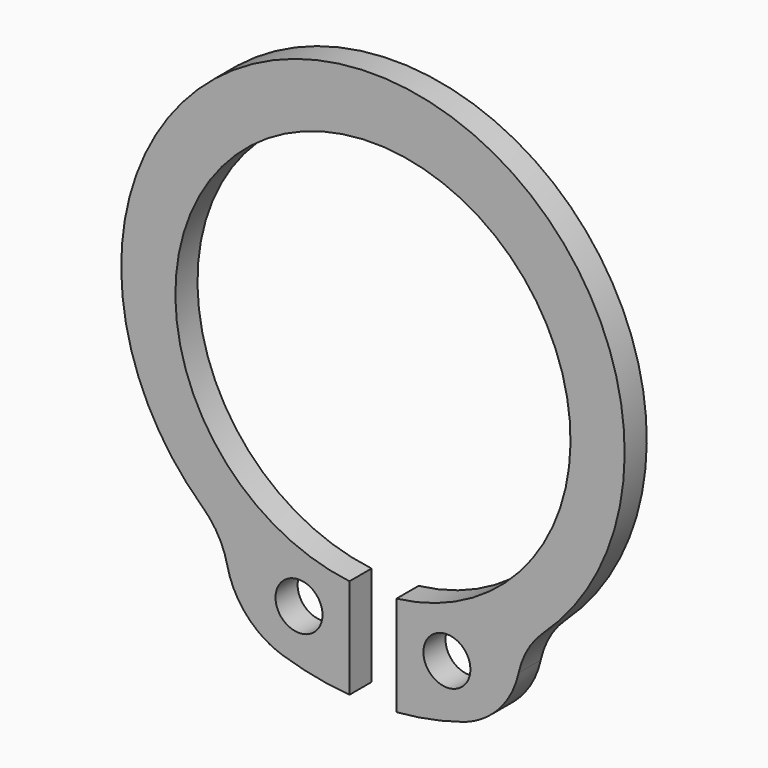
from build123d import *

# Parameters (mm, degrees)
F0_R        = 0.85
F1_DEPTH    = 1
F2_T1_DEPTH = 1
F3_R        = 3


# Not quite as in the source:
# - a fillet or chamfer that OpenCascade refuses, or shapes differently, is made with other operations: its cross-section is extruded or revolved along the edge and cut away or added


with BuildPart() as f1:
    # F0 (on Front) → F1 (new body)
    with BuildSketch(Plane.XZ):
        with BuildLine():
            ThreePointArc((-0.85, -7.0992957397), (0, 7.15), (0.85, -7.0992957397))
            Line((0.85, -7.0992957397), (0.85, -10.7163426597))
            ThreePointArc((0.85, -10.7163426597), (3.1412802118, -10.2808004859), (5.2846966911, -9.3613290127))
            Line((5.2846966911, -9.3613290127), (4.5, -7.6785415282))
            ThreePointArc((4.5, -7.6785415282), (0, 9.3500403242), (-4.5, -7.6785415282))
            Line((-4.5, -7.6785415282), (-5.2846966911, -9.3613290127))
            ThreePointArc((-5.2846966911, -9.3613290127), (-3.1412802118, -10.2808004859), (-0.85, -10.7163426597))
            Line((-0.85, -10.7163426597), (-0.85, -7.0992957397))
        make_face()
        with Locations((-2.6762816156, -8.4880808617)):
            Circle(F0_R, mode=Mode.SUBTRACT)
        with Locations((2.6762816156, -8.4880808617)):
            Circle(F0_R, mode=Mode.SUBTRACT)
    extrude(amount=F1_DEPTH)

    # F2: fillet of radius 3 on 2 edges, made by hand

    # F2_s2 → F2_t1 (join)
    with BuildSketch(Plane.XZ):
        with BuildLine():
            ThreePointArc((-6.170677683, -6.4591691909), (-5.3337110531, -7.7899747588), (-5.2846966911, -9.3613290127))
            Line((-5.2846966911, -9.3613290127), (-4.5, -7.6785415282))
            ThreePointArc((-4.5, -7.6785415282), (-5.3700612452, -7.1164289704), (-6.170677683, -6.4591691909))
        make_face()
        with BuildLine():
            ThreePointArc((5.2846966911, -9.3613290127), (5.3337110531, -7.7899747588), (6.170677683, -6.4591691909))
            ThreePointArc((6.170677683, -6.4591691909), (5.3700612452, -7.1164289704), (4.5, -7.6785415282))
            Line((4.5, -7.6785415282), (5.2846966911, -9.3613290127))
        make_face()
    extrude(amount=F2_T1_DEPTH)

    # F3
    f3_edges = [f1.edges().sort_by_distance(p)[0] for p in [
        (-5.284697, -0.5, -9.361329),
        (5.284697, -0.5, -9.361329),
    ]]
    fillet(f3_edges, radius=F3_R)


solid = f1.part
